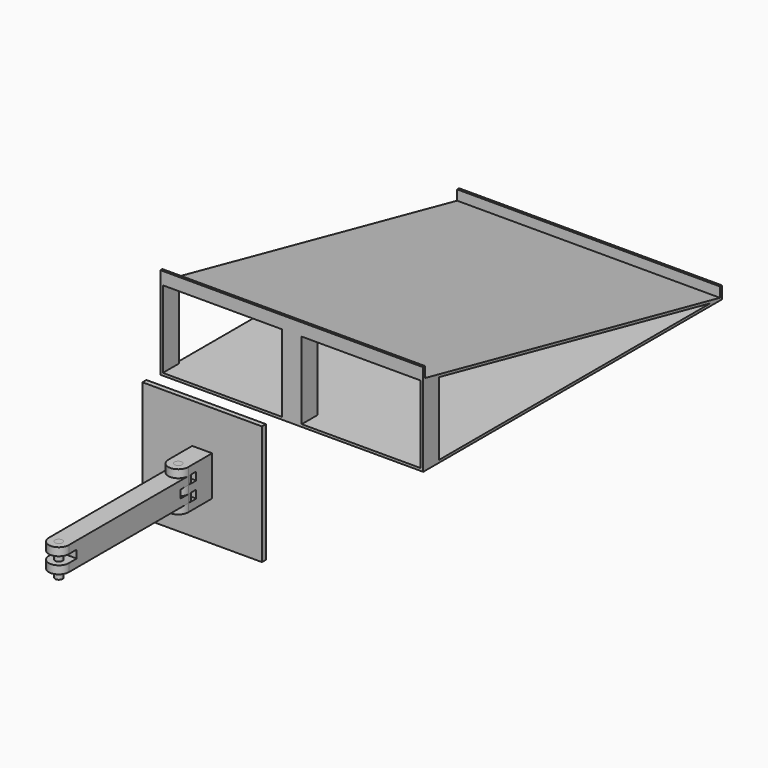
from build123d import *

# Parameters (mm, degrees)
F0_W          = 76.2
F0_H          = 76.2
F1_DEPTH      = 3.175
F2_W          = 12.7
F2_H          = 19.05
F3_DEPTH      = 12.7
F4_W          = 12.7
F4_H          = 5.08
F5_DEPTH      = 38.101
F5_DEPTH_BACK = 38.101
F6_W          = 12.7
F6_H          = 19.05
F7_DEPTH      = 7.62
F8_W          = 6.35
F8_H          = 5.08
F9_DEPTH      = 25.4
F10_R         = 2.38125
F11_DEPTH     = 50.801
F12_DEPTH     = 76.2
F14_DEPTH     = 15.24
F15_W         = 6.35
F15_H         = 5.08
F16_DEPTH     = 44.451
F17_R         = 2.38125
F18_DEPTH     = 45.721
F19_W         = 12.7
F19_H         = 12.7
F20_DEPTH     = 50.8
F22_DEPTH     = 44.451
F23_W         = 1.5875
F23_H         = 6.35
F24_DEPTH     = 83.82
F26_DEPTH     = 1.5875
F28_DEPTH     = 1.5875
F29_R         = 2.38125
F30_DEPTH     = 25.4
F31_R         = 2.38125
F32_DEPTH     = 20.32


with BuildPart() as f1:
    # F0 (on Front) → F1 (new body)
    with BuildSketch(Plane.XZ):
        Rectangle(F0_W, F0_H)
    extrude(amount=F1_DEPTH)


with BuildPart() as f3:
    # F2 (on Top) → F3 (new body, symmetric)
    with BuildSketch(Plane.XY):
        with Locations((0, -12.7)):
            Rectangle(F2_W, F2_H)
        with BuildLine():
            ThreePointArc((-6.35, -22.225), (0, -28.575), (6.35, -22.225))
            Line((6.35, -22.225), (-6.35, -22.225))
        make_face()
    extrude(amount=F3_DEPTH, both=True)

    # F4 (on Right) → F5 (cut, two sides)
    with BuildSketch(Plane.YZ) as f5_sk:
        with Locations((-22.225, 5.08)):
            Rectangle(F4_W, F4_H)
        with Locations((-22.225, -5.08)):
            Rectangle(F4_W, F4_H)
    extrude(amount=-F5_DEPTH, mode=Mode.SUBTRACT)
    extrude(f5_sk.sketch, amount=F5_DEPTH_BACK, mode=Mode.SUBTRACT)


with BuildPart() as f7:
    # F6 (on Top) → F7 (new body, symmetric)
    with BuildSketch(Plane.XY):
        with BuildLine():
            Line((-6.35, -22.225), (6.35, -22.225))
            ThreePointArc((6.35, -22.225), (0, -15.875), (-6.35, -22.225))
        make_face()
        with Locations((0, -31.75)):
            Rectangle(F6_W, F6_H)
    extrude(amount=F7_DEPTH, both=True)

    # F8 (on face) → F9 (cut)
    with BuildSketch(Plane.YZ.offset(6.35)):
        Polygon((-3.175, 12.7), (-22.225, 12.7), (-22.225, 7.62), (-15.875, 7.62), (-15.875, 2.54), (-22.225, 2.54), (-22.225, -2.54), (-15.875, -2.54), (-15.875, -7.62), (-22.225, -7.62), (-22.225, -12.7), (-3.175, -12.7), align=None)
        with Locations((-25.4, 0)):
            Rectangle(F8_W, F8_H)
    extrude(amount=-F9_DEPTH, mode=Mode.SUBTRACT)


with BuildPart() as f11_tool:
    # F10 (on face) → F11 (new body, through all)
    with BuildSketch(Plane.XY.offset(12.7)):
        with Locations((0, -22.225)):
            Circle(F10_R)
    extrude(amount=-F11_DEPTH)


with BuildPart() as f3_1:
    add(f3.part)

    # F11: cut by f11_tool
    add(f11_tool.part, mode=Mode.SUBTRACT)


with BuildPart() as f7_1:
    add(f7.part)

    # F11: cut by f11_tool
    add(f11_tool.part, mode=Mode.SUBTRACT)

    # F12 (add): a face of the model
    f12_faces = [f7_1.faces().sort_by_distance(p)[0] for p in [
        (0, -41.275, 0),
    ]]
    extrude(f12_faces, amount=F12_DEPTH)

    # F13 (on face) → F14 (join)
    with BuildSketch(Plane.XY.offset(7.62)):
        with BuildLine():
            Line((6.35, -117.475), (-6.35, -117.475))
            ThreePointArc((-6.35, -117.475), (0, -123.825), (6.35, -117.475))
        make_face()
    extrude(amount=-F14_DEPTH)

    # F15 (on face) → F16 (cut, through all)
    with BuildSketch(Plane.YZ.offset(6.35)):
        with Locations((-120.65, 0)):
            Rectangle(F15_W, F15_H)
        with Locations((-114.3, 0)):
            Rectangle(F15_W, F15_H)
    extrude(amount=-F16_DEPTH, mode=Mode.SUBTRACT)

    # F17 (on face) → F18 (cut, through all)
    with BuildSketch(Plane.XY.offset(7.62)):
        with Locations((0, -117.475)):
            Circle(F17_R)
    extrude(amount=-F18_DEPTH, mode=Mode.SUBTRACT)


with BuildPart() as f20:
    # F19 (on Top) → F20 (new body)
    with BuildSketch(Plane.XY):
        with Locations((0, 74.602655525)):
            Rectangle(F19_W, F19_H)
    extrude(amount=F20_DEPTH)

    # F21 (on face) → F22 (cut, through all)
    with BuildSketch(Plane.YZ.offset(6.35)):
        Polygon((68.252655525, 56.2568344176), (68.252655525, 50.8), (80.952655525, 48.0725299054), (81.430234015, 56.2568344176), align=None)
    extrude(amount=-F22_DEPTH, mode=Mode.SUBTRACT)

    # F23 (on Right) → F24 (join, symmetric)
    with BuildSketch(Plane.YZ):
        Polygon((297.2337353981, 0), (68.252655525, 0), (68.252655525, -1.5875), (306.3817041481, -1.5875), (306.3817041481, 0), (304.7942041481, 0), align=None)
        Polygon((68.252655525, 49.1763029593), (297.2337353981, 0), (304.7942041481, 0), (69.840155525, 50.4590662382), (68.252655525, 50.8), align=None)
        with Locations((305.5879541481, 3.175)):
            Rectangle(F23_W, F23_H)
        Polygon((68.252655525, 50.8), (69.840155525, 50.4590662382), (69.840155525, 57.15), (68.252655525, 57.15), align=None)
    extrude(amount=F24_DEPTH, both=True)

    # F25 (on face) → F26 (join)
    with BuildSketch(Plane.YZ.offset(83.82)):
        Polygon((80.952655525, 0), (80.952655525, 46.4488328647), (68.252655525, 49.1763029593), (68.252655525, 0), align=None)
    extrude(amount=-F26_DEPTH)

    # F27 (on face) → F28 (join)
    with BuildSketch(Plane(origin=(-83.82, 0, 0), x_dir=(0, -1, 0), z_dir=(-1, 0, 0))):
        Polygon((-80.952655525, 0), (-68.252655525, 0), (-68.252655525, 49.1763029593), (-80.952655525, 46.4488328647), align=None)
    extrude(amount=-F28_DEPTH)


with BuildPart() as f30:
    # F29 (on face) → F30 (new body)
    with BuildSketch(Plane.XY.offset(12.7)):
        with Locations((0, -22.225)):
            Circle(F29_R)
    extrude(amount=-F30_DEPTH)


with BuildPart() as f32:
    # F31 (on face) → F32 (new body)
    with BuildSketch(Plane.XY.offset(7.62)):
        with Locations((0, -117.475)):
            Circle(F31_R)
    extrude(amount=-F32_DEPTH)


solid = Compound([f1.part, f3_1.part, f7_1.part, f20.part, f30.part, f32.part])
